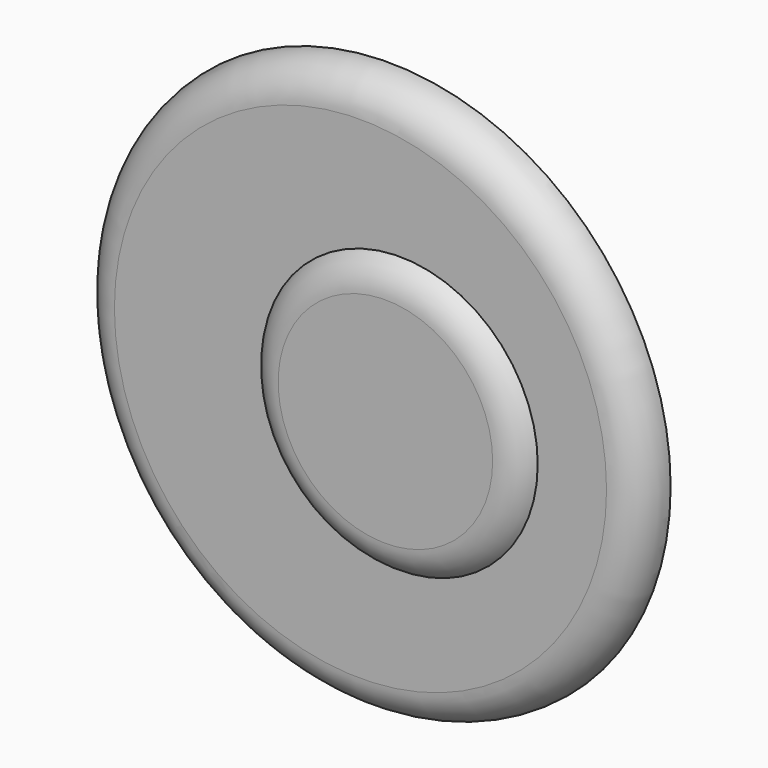
from build123d import *

# Parameters (mm, degrees)
F0_R     = 40.1789827743
F1_DEPTH = 5.08
F2_R     = 19.6940122024
F3_DEPTH = 2.54
F4_R     = 5.07999


# Not quite as in the source:
# - a fillet or chamfer that OpenCascade refuses, or shapes differently, is made with other operations: its cross-section is extruded or revolved along the edge and cut away or added
# - a fillet or chamfer is up to 0.001 mm smaller than in the source, because OpenCascade refuses the exact size


with BuildPart() as f1:
    # F0 (on Front) → F1 (new body)
    with BuildSketch(Plane.XZ):
        Circle(F0_R)
    extrude(amount=F1_DEPTH)

    # F2 (on face) → F3 (join)
    with BuildSketch(Plane.XZ.offset(5.08)):
        with Locations((5.5896993726, 0)):
            Circle(F2_R)
    extrude(amount=F3_DEPTH)

    # F4 (radius 5.08 in the source; OpenCascade refuses exactly that, so slightly less here)
    f4_edges = [f1.edges().sort_by_distance(p)[0] for p in [
        (-40.178983, -5.08, 0),
    ]]
    fillet(f4_edges, radius=F4_R)

    # F5: fillet of radius 5.08 on 1 edges, made by hand

    # F5_s1 → F5_t2 (revolve, cut)
    with BuildSketch(Plane.XY):
        with BuildLine():
            ThreePointArc((25.283711575, -5.08), (23.4243025238, -6.9394090512), (20.8843025238, -7.62))
            Line((20.8843025238, -7.62), (25.283711575, -7.62))
            Line((25.283711575, -7.62), (25.283711575, -5.08))
        make_face()
    revolve(axis=Axis((5.5896993726, -7.62, 0), (0, -1, 0)), mode=Mode.SUBTRACT)


solid = f1.part
